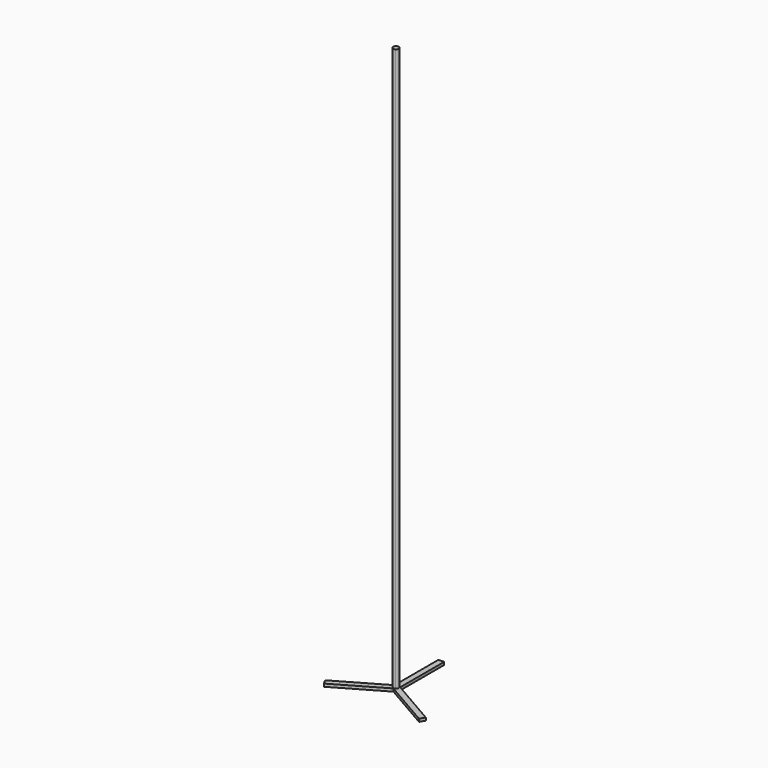
from build123d import *

# Parameters (mm, degrees)
F1_DEPTH = 5
F2_DEPTH = 1000


with BuildPart() as f1:
    # F0 (on Top) → F1 (new body)
    with BuildSketch(Plane.XY):
        with BuildLine():
            Line((-5, 100), (-5, 2.8867513459))
            Line((-5, 2.8867513459), (-2.5, 4.3301270189))
            ThreePointArc((-2.5, 4.3301270189), (0, 5), (2.5, 4.3301270189))
            Line((2.5, 4.3301270189), (5, 2.8867513459))
            Line((5, 2.8867513459), (5, 100))
            Line((5, 100), (-5, 100))
        make_face()
        with BuildLine():
            Line((-2.5, 4.3301270189), (-5, 2.8867513459))
            Line((-5, 2.8867513459), (-5, 0))
            ThreePointArc((-5, 0), (-4.3301270189, 2.5), (-2.5, 4.3301270189))
        make_face()
        with BuildLine():
            Line((-89.1025403784, -45.6698729811), (-86.6025403784, -50))
            Line((-86.6025403784, -50), (-84.1025403784, -54.3301270189))
            Line((-84.1025403784, -54.3301270189), (0, -5.7735026919))
            Line((0, -5.7735026919), (-2.5, -4.3301270189))
            ThreePointArc((-2.5, -4.3301270189), (-4.3301270189, -2.5), (-5, 0))
            Line((-5, 0), (-5, 2.8867513459))
            Line((-5, 2.8867513459), (-89.1025403784, -45.6698729811))
        make_face()
        with BuildLine():
            Line((-2.5, -4.3301270189), (0, -5.7735026919))
            Line((0, -5.7735026919), (2.5, -4.3301270189))
            ThreePointArc((2.5, -4.3301270189), (0, -5), (-2.5, -4.3301270189))
        make_face()
        with BuildLine():
            Line((2.5, -4.3301270189), (0, -5.7735026919))
            Line((0, -5.7735026919), (84.1025403784, -54.3301270189))
            Line((84.1025403784, -54.3301270189), (86.6025403784, -50))
            Line((86.6025403784, -50), (89.1025403784, -45.6698729811))
            Line((89.1025403784, -45.6698729811), (5, 2.8867513459))
            Line((5, 2.8867513459), (5, 0))
            ThreePointArc((5, 0), (4.3301270189, -2.5), (2.5, -4.3301270189))
        make_face()
        with BuildLine():
            Line((5, 2.8867513459), (2.5, 4.3301270189))
            ThreePointArc((2.5, 4.3301270189), (4.3301270189, 2.5), (5, 0))
            Line((5, 0), (5, 2.8867513459))
        make_face()
    extrude(amount=F1_DEPTH)

    # F0 (on Top) → F2 (join)
    with BuildSketch(Plane.XY):
        with BuildLine():
            Line((2.5, 4.3301270189), (0, 0))
            Line((0, 0), (5, 0))
            ThreePointArc((5, 0), (4.3301270189, 2.5), (2.5, 4.3301270189))
        make_face()
        with BuildLine():
            Line((0, 0), (2.5, -4.3301270189))
            ThreePointArc((2.5, -4.3301270189), (4.3301270189, -2.5), (5, 0))
            Line((5, 0), (0, 0))
        make_face()
        with BuildLine():
            ThreePointArc((-2.5, -4.3301270189), (0, -5), (2.5, -4.3301270189))
            Line((2.5, -4.3301270189), (0, 0))
            Line((0, 0), (-2.5, -4.3301270189))
        make_face()
        with BuildLine():
            Line((0, 0), (-5, 0))
            ThreePointArc((-5, 0), (-4.3301270189, -2.5), (-2.5, -4.3301270189))
            Line((-2.5, -4.3301270189), (0, 0))
        make_face()
        with BuildLine():
            Line((0, 0), (-2.5, 4.3301270189))
            ThreePointArc((-2.5, 4.3301270189), (-4.3301270189, 2.5), (-5, 0))
            Line((-5, 0), (0, 0))
        make_face()
        with BuildLine():
            ThreePointArc((2.5, 4.3301270189), (0, 5), (-2.5, 4.3301270189))
            Line((-2.5, 4.3301270189), (0, 0))
            Line((0, 0), (2.5, 4.3301270189))
        make_face()
    extrude(amount=F2_DEPTH)


solid = f1.part
